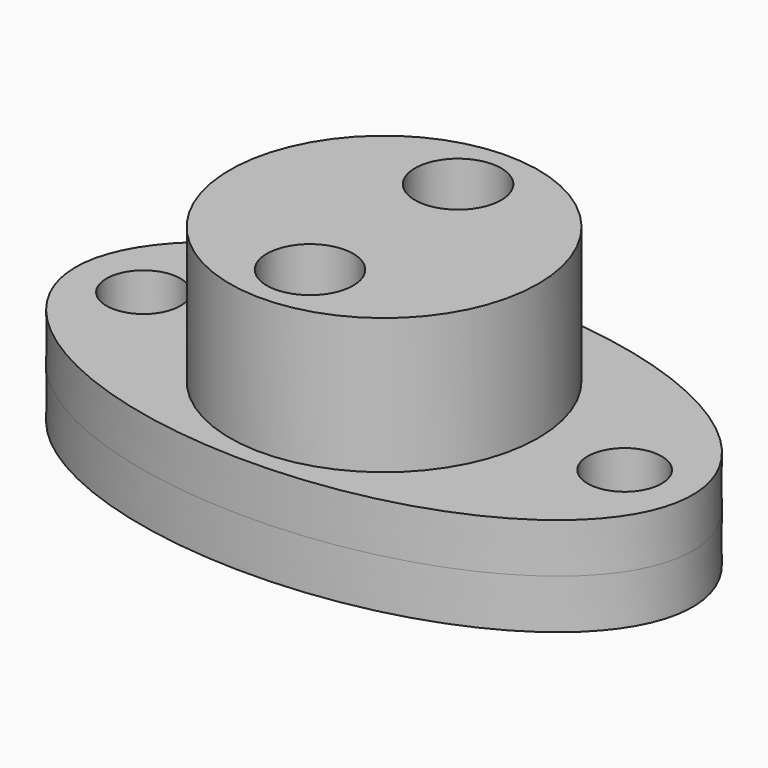
from build123d import *

# Parameters (mm, degrees)
F0_R      = 3
F1_DEPTH  = 8
F0_R_2    = 12.5
F0_R_3    = 3.5
F2_DEPTH  = 15
F4_DEPTH  = 4
F5_R      = 3
F6_DEPTH  = 10
F8_R      = 1.75
F9_DEPTH  = 10
F10_R     = 1.75
F11_DEPTH = 10
F12_R     = 1.75
F13_DEPTH = 10
F14_R     = 1.75
F15_DEPTH = 10
F7_R      = 1.75
F7_R_2    = 3
F17_DEPTH = 4
F19_DEPTH = 5


with BuildPart() as f1:
    # F0 (on Top) → F1 (new body)
    with BuildSketch(Plane.XY):
        with Locations((0, 7.5)):
            Circle(F0_R)
    extrude(amount=F1_DEPTH)

    # F12 (on face) → F13 (cut)
    with BuildSketch(Plane(origin=(0, 0, 0), x_dir=(1, 0, 0), z_dir=(0, 0, -1))):
        with Locations((0, -7.5)):
            Circle(F12_R)
    extrude(amount=-F13_DEPTH, mode=Mode.SUBTRACT)


with BuildPart() as f1b:
    # F0 (on Top) → F1, piece 2 (new body)
    with BuildSketch(Plane.XY):
        with Locations((0, -7.5)):
            Circle(F0_R)
    extrude(amount=F1_DEPTH)

    # F14 (on face) → F15 (cut)
    with BuildSketch(Plane(origin=(0, 0, 0), x_dir=(1, 0, 0), z_dir=(0, 0, -1))):
        with Locations((0, 7.5)):
            Circle(F14_R)
    extrude(amount=-F15_DEPTH, mode=Mode.SUBTRACT)


with BuildPart() as f2:
    # F0 (on Top) → F2 (new body)
    with BuildSketch(Plane.XY):
        Circle(F0_R_2)
        with Locations((0, -7.5)):
            Circle(F0_R_3, mode=Mode.SUBTRACT)
        with Locations((0, 7.5)):
            Circle(F0_R_3, mode=Mode.SUBTRACT)
    extrude(amount=F2_DEPTH)


with BuildPart() as f4:
    # F3 (on face) → F4 (new body)
    with BuildSketch(Plane(origin=(0, 0, 0), x_dir=(1, 0, 0), z_dir=(0, 0, -1))):
        with BuildLine():
            Line((-25, 0), (0, 0))
            Line((0, 0), (0, 14))
            add(Edge.make_bspline(
                [(0, 14), (-25, 14), (-25, 0)],
                knots=[1.5707963268, 1.5707963268, 1.5707963268, 3.1415926536, 3.1415926536, 3.1415926536], degree=2, weights=[1, 0.7071067812, 1]))
        make_face()
        with BuildLine():
            Line((0, -14), (0, 0))
            Line((0, 0), (-25, 0))
            add(Edge.make_bspline(
                [(-25, 0), (-25, -14), (0, -14)],
                knots=[3.1415926536, 3.1415926536, 3.1415926536, 4.7123889804, 4.7123889804, 4.7123889804], degree=2, weights=[1, 0.7071067812, 1]))
        make_face()
        with BuildLine():
            Line((0, 14), (0, 0))
            Line((0, 0), (25, 0))
            add(Edge.make_bspline(
                [(25, 0), (25, 14), (0, 14)],
                knots=[0, 0, 0, 1.5707963268, 1.5707963268, 1.5707963268], degree=2, weights=[1, 0.7071067812, 1]))
        make_face()
        with BuildLine():
            Line((25, 0), (0, 0))
            Line((0, 0), (0, -14))
            add(Edge.make_bspline(
                [(0, -14), (25, -14), (25, 0)],
                knots=[4.7123889804, 4.7123889804, 4.7123889804, 6.2831853072, 6.2831853072, 6.2831853072], degree=2, weights=[1, 0.7071067812, 1]))
        make_face()
    extrude(amount=-F4_DEPTH)

    # F5 (on face) → F6 (cut)
    with BuildSketch(Plane(origin=(0, 0, 0), x_dir=(1, 0, 0), z_dir=(0, 0, -1))):
        with Locations((-19.5, 0)):
            Circle(F5_R)
        with Locations((19.5, 0)):
            Circle(F5_R)
    extrude(amount=-F6_DEPTH, mode=Mode.SUBTRACT)

    # F8 (on face) → F9 (cut)
    with BuildSketch(Plane.XY.offset(8)):
        with Locations((0, 7.5)):
            Circle(F8_R)
    extrude(amount=-F9_DEPTH, mode=Mode.SUBTRACT)

    # F10 (on face) → F11 (cut)
    with BuildSketch(Plane.XY.offset(8)):
        with Locations((0, -7.5)):
            Circle(F10_R)
    extrude(amount=-F11_DEPTH, mode=Mode.SUBTRACT)


with BuildPart() as f17:
    # F7 (on face) → F17 (new body)
    with BuildSketch(Plane(origin=(0, 0, 0), x_dir=(1, 0, 0), z_dir=(0, 0, -1))):
        with BuildLine():
            add(Edge.make_bspline(
                [(0, -14), (7.0710678119, -14), (15.716991411, -12.5502525317), (22.4111652352, -8.8015151902), (25, -3.9597979746), (25, 3.9597979746), (22.4111652352, 8.8015151902), (15.716991411, 12.5502525317), (7.0710678119, 14), (-7.0710678119, 14), (-15.716991411, 12.5502525317), (-22.4111652352, 8.8015151902), (-25, 3.9597979746), (-25, -3.9597979746), (-22.4111652352, -8.8015151902), (-15.716991411, -12.5502525317), (-7.0710678119, -14), (0, -14)],
                knots=[4.7123889804, 4.7123889804, 4.7123889804, 4.7123889804, 4.7123889804, 4.7123889804, 6.2831853072, 6.2831853072, 6.2831853072, 6.2831853072, 7.853981634, 7.853981634, 7.853981634, 7.853981634, 9.4247779608, 9.4247779608, 9.4247779608, 9.4247779608, 10.9955742876, 10.9955742876, 10.9955742876, 10.9955742876, 10.9955742876, 10.9955742876], degree=5, weights=[1, 1, 0.9656854249, 0.9656854249, 1, 1, 0.9656854249, 0.9656854249, 1, 1, 0.9656854249, 0.9656854249, 1, 1, 0.9656854249, 0.9656854249, 1, 1]))
        make_face()
        with Locations((0, -7.5)):
            Circle(F7_R, mode=Mode.SUBTRACT)
        with Locations((-19.5, 0)):
            Circle(F7_R_2, mode=Mode.SUBTRACT)
        with Locations((19.5, 0)):
            Circle(F7_R_2, mode=Mode.SUBTRACT)
        with Locations((0, 7.5)):
            Circle(F7_R, mode=Mode.SUBTRACT)
    extrude(amount=F17_DEPTH)

    # F18 (on face) → F19 (cut)
    with BuildSketch(Plane(origin=(0, 0, -4), x_dir=(1, 0, 0), z_dir=(0, 0, -1))):
        with BuildLine():
            ThreePointArc((3.5, 7.5), (-2.4748737342, 9.9748737342), (0, 4))
            ThreePointArc((0, 4), (2.4748737342, 5.0251262658), (3.5, 7.5))
        make_face()
        with BuildLine():
            ThreePointArc((3.5, -7.5), (2.4748737342, -5.0251262658), (0, -4))
            ThreePointArc((0, -4), (-2.4748737342, -9.9748737342), (3.5, -7.5))
        make_face()
    extrude(amount=-F19_DEPTH, mode=Mode.SUBTRACT)


solid = Compound([f1.part, f1b.part, f2.part, f4.part, f17.part])
